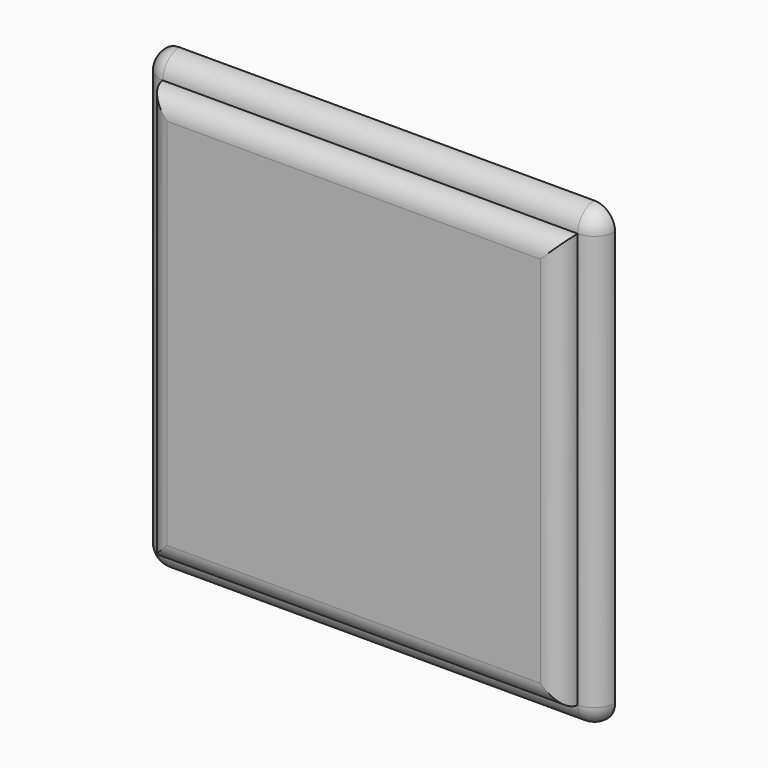
from build123d import *

# Parameters (mm, degrees)
F0_W     = 100
F0_H     = 100
F1_DEPTH = 5
F2_W     = 110
F2_H     = 110
F3_DEPTH = 5
F4_R     = 5
F5_R     = 4.99999
F6_R     = 4.99999


# Not quite as in the source:
# - a fillet or chamfer is up to 0.001 mm smaller than in the source, because OpenCascade refuses the exact size


with BuildPart() as f1:
    # F0 (on Front) → F1 (new body)
    with BuildSketch(Plane.XZ):
        Rectangle(F0_W, F0_H)
    extrude(amount=F1_DEPTH)

    # F2 (on face) → F3 (join)
    with BuildSketch(Plane(origin=(0, 0, 0), x_dir=(-1, 0, 0), z_dir=(0, 1, 0))):
        Rectangle(F2_W, F2_H)
    extrude(amount=F3_DEPTH)

    # F4
    f4_edges = [f1.edges().sort_by_distance(p)[0] for p in [
        (-55, 2.5, -55),
        (55, 2.5, -55),
        (55, 2.5, 55),
        (-55, 2.5, 55),
    ]]
    fillet(f4_edges, radius=F4_R)

    # F5 (radius 5 in the source; OpenCascade refuses exactly that, so slightly less here)
    f5_edges = [f1.edges().sort_by_distance(p)[0] for p in [
        (0, -5, 50),
        (50, -5, 0),
        (0, -5, -50),
        (-50, -5, 0),
    ]]
    fillet(f5_edges, radius=F5_R)

    # F6 (radius 5 in the source; OpenCascade refuses exactly that, so slightly less here)
    f6_edges = [f1.edges().sort_by_distance(p)[0] for p in [
        (0, 0, -55),
    ]]
    fillet(f6_edges, radius=F6_R)


solid = f1.part
